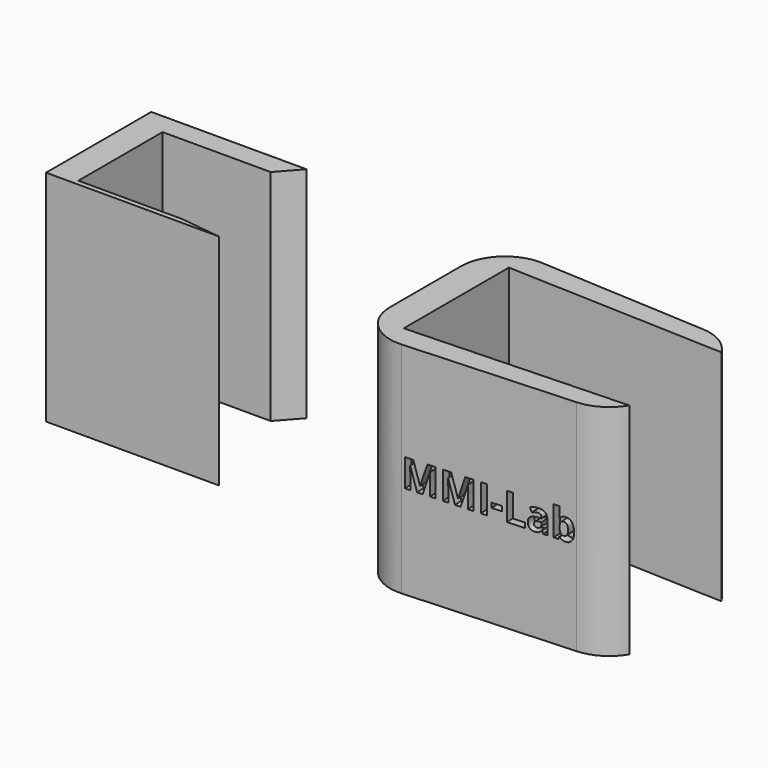
from build123d import *

# Parameters (mm, degrees)
F1_DEPTH     = 25
F2_T1_DEPTH  = 51.385064932
F2_T3_DEPTH  = 72.7662185931
F3_TEXT_SIZE = 4.4041950734
F4_DEPTH     = 1


# Not quite as in the source:
# - a fillet or chamfer that OpenCascade refuses, or shapes differently, is made with other operations: its cross-section is extruded or revolved along the edge and cut away or added
# - Text() gives the source's letters only with a copy of the font that has no kerning and outlines rounded to 1/6400 em; it was checked with that copy


with BuildPart() as f1:
    # F0 (on Top) → F1 (new body)
    with BuildSketch(Plane.XY):
        Polygon((-24.4529437022, 8.6368946359), (-12.117555365, 8.6368946359), (-9.972397238, 11.0501972958), (-27.6699513197, 11.0501972958), (-27.6699513197, -3.9498027042), (-7.9613104463, -3.9498027042), (-12.653844431, -3.3631053641), (-24.4529437022, -3.3631053641), align=None)
    extrude(amount=F1_DEPTH)


with BuildPart() as f1b:
    # F0 (on Top) → F1, piece 2 (new body)
    with BuildSketch(Plane.XY):
        Polygon((12.458268553, 10.3333480603), (12.458268553, 0), (12.458268553, -10.3333480603), (46.4427731931, -8.499937132), (40.9406697408, -6.5621136048), (15.958268553, -7.5), (15.958268553, 0), (15.958268553, 7.5), (40.9406697408, 6.5621136048), (46.4427731931, 8.499937132), align=None)
    extrude(amount=F1_DEPTH)

    # F2: fillet of radius 5 on 4 edges, made by hand

    # F2_s2 → F2_t1 (cut)
    with BuildSketch(Plane.XY.offset(-13.192532466)):
        with BuildLine():
            ThreePointArc((12.458268553, 5.0563350739), (14.0192826957, 8.6858496796), (17.7276190624, 10.0490748331))
            Line((17.7276190624, 10.0490748331), (12.458268553, 10.3333480603))
            Line((12.458268553, 10.3333480603), (12.458268553, 5.0563350739))
        make_face()
        with BuildLine():
            ThreePointArc((12.458268553, -5.0563350739), (14.0192826957, -8.6858496796), (17.7276190624, -10.0490748331))
            Line((17.7276190624, -10.0490748331), (12.458268553, -10.3333480603))
            Line((12.458268553, -10.3333480603), (12.458268553, -5.0563350739))
        make_face()
    extrude(amount=F2_T1_DEPTH, mode=Mode.SUBTRACT)

    # F2_s4 → F2_t3 (cut)
    with BuildSketch(Plane.XY.offset(-23.8831092966)):
        with BuildLine():
            ThreePointArc((40.9406697408, 6.5621136048), (39.2299150405, 8.2951778745), (36.9034012445, 9.0145713444))
            Line((36.9034012445, 9.0145713444), (46.4427731931, 8.499937132))
            Line((46.4427731931, 8.499937132), (40.9406697408, 6.5621136048))
        make_face()
        with BuildLine():
            ThreePointArc((40.9406697408, -6.5621136048), (39.2299150405, -8.2951778745), (36.9034012445, -9.0145713444))
            Line((36.9034012445, -9.0145713444), (46.4427731931, -8.499937132))
            Line((46.4427731931, -8.499937132), (40.9406697408, -6.5621136048))
        make_face()
    extrude(amount=F2_T3_DEPTH, mode=Mode.SUBTRACT)


with BuildPart() as f4:
    # F3 (on face) → F4 (new body)
    with BuildSketch(Plane(origin=(0.5920039621, -10.9735144952, 0), x_dir=(0.9985479518, 0.0538701019, 0), z_dir=(0.0538701019, -0.9985479518, 0))):
        with Locations((17.1605330207, 10.66040006)):
            Text('MMI-Lab', F3_TEXT_SIZE, font='Open Sans', font_style=FontStyle.BOLD, text_align=(TextAlign.LEFT, TextAlign.BOTTOM))
    extrude(amount=-F4_DEPTH)


with BuildPart() as f1b_1:
    add(f1b.part)

    # F5: cut F4
    add(f4.part, mode=Mode.SUBTRACT)


solid = Compound([f1.part, f1b_1.part])
